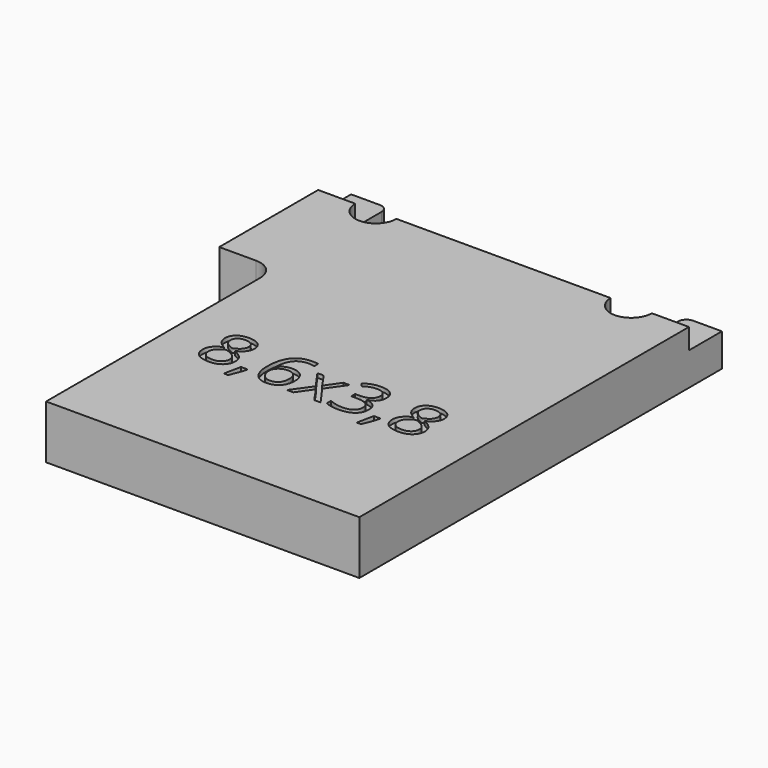
from build123d import *

# Parameters (mm, degrees)
F1_DEPTH     = 13
F2_W         = 107.3082715438
F2_H         = 14.5000026375
F3_DEPTH     = 5
F4_R         = 3
F5_DEPTH     = 10
F6_TEXT_SIZE = 16.861082986
F7_DEPTH     = 1


# Not quite as in the source:
# - Text() gives the source's letters only with a copy of the font that has no kerning and outlines rounded to 1/6400 em; it was checked with that copy


with BuildPart() as f1:
    # F0 (on Top) → F1 (new body)
    with BuildSketch(Plane.XY):
        with BuildLine():
            Line((-41.4800007343, 29.9199996144), (-41.4800007343, -10.0800003856))
            Line((-41.4800007343, -10.0800003856), (-32.5100003928, -10.0800003856))
            ThreePointArc((-32.5100003928, -10.0800003856), (-28.9744664869, -11.5444664797), (-27.5100003928, -15.0800003856))
            Line((-27.5100003928, -15.0800003856), (-27.5100003928, -80.0800003856))
            Line((-27.5100003928, -80.0800003856), (48.5199992657, -80.0800003856))
            Line((48.5199992657, -80.0800003856), (48.5199992657, 29.9199996144))
            Line((48.5199992657, 29.9199996144), (41.5199992657, 29.9199996144))
            ThreePointArc((41.5199992657, 29.9199996144), (40.1057857033, 29.3342131767), (39.5199992657, 27.9199996144))
            Line((39.5199992657, 27.9199996144), (39.5199992657, 19.9199996144))
            ThreePointArc((39.5199992657, 19.9199996144), (34.5199992657, 14.9199996144), (29.5199992657, 19.9199996144))
            Line((29.5199992657, 19.9199996144), (-22.4800007343, 19.9199996144))
            ThreePointArc((-22.4800007343, 19.9199996144), (-27.4800007343, 14.9199996144), (-32.4800007343, 19.9199996144))
            Line((-32.4800007343, 19.9199996144), (-32.4800007343, 27.9199996144))
            ThreePointArc((-32.4800007343, 27.9199996144), (-33.065787172, 29.3342131767), (-34.4800007343, 29.9199996144))
            Line((-34.4800007343, 29.9199996144), (-41.4800007343, 29.9199996144))
        make_face()
    extrude(amount=F1_DEPTH)

    # F2 (on face) → F3 (cut)
    with BuildSketch(Plane.XY.offset(13)):
        with Locations((10.5722389322, 27.1700009331)):
            Rectangle(F2_W, F2_H)
    extrude(amount=-F3_DEPTH, mode=Mode.SUBTRACT)

    # F4 (on face) → F5 (cut)
    with BuildSketch(Plane(origin=(0, 19.9199996144, 0), x_dir=(-1, 0, 0), z_dir=(0, 1, 0))):
        with Locations((-3.5199992657, 6.5)):
            Circle(F4_R)
    extrude(amount=-F5_DEPTH, mode=Mode.SUBTRACT)

    # F6 (on face) → F7 (cut)
    with BuildSketch(Plane.XY.offset(13)):
        with Locations((-18.5406059027, -47.8933230042)):
            Text('8,6x3,8', F6_TEXT_SIZE, font='Open Sans', text_align=(TextAlign.LEFT, TextAlign.BOTTOM))
    extrude(amount=-F7_DEPTH, mode=Mode.SUBTRACT)


solid = f1.part
